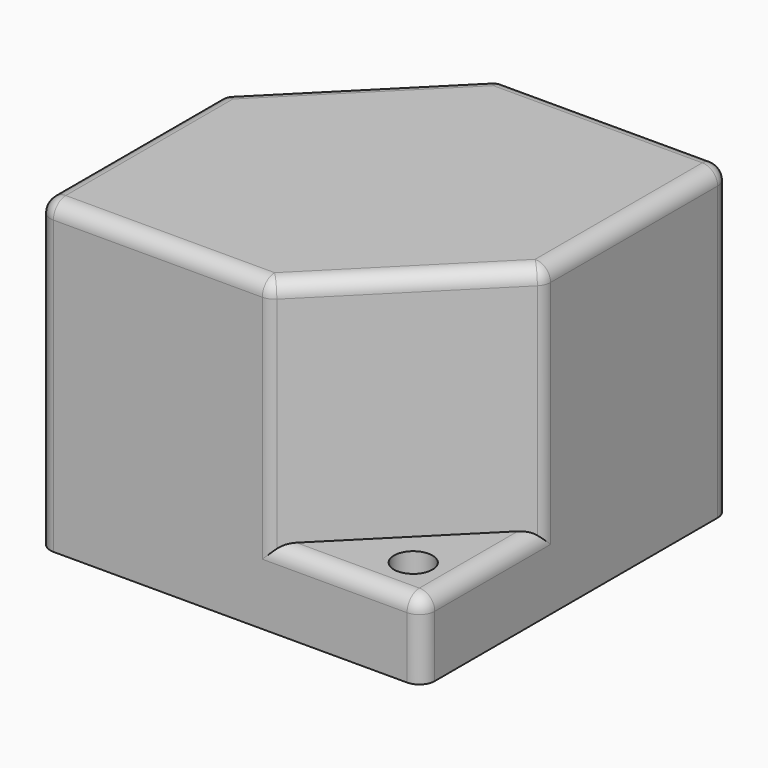
from build123d import *

# Parameters (mm, degrees)
F0_W     = 127
F0_H     = 127
F1_DEPTH = 101.6
F3_DEPTH = 76.2
F4_R     = 6.35
F5_DEPTH = 203.2
F6_T     = -2.54
F7_R     = 5.08


# Not quite as in the source:
# - a feature names something its author has since deleted; it is built from what else it names


with BuildPart() as f1:
    # F0 (on Top) → F1 (new body)
    with BuildSketch(Plane.XY):
        with Locations((2.0048860461, 1.4262827701)):
            Rectangle(F0_W, F0_H)
    extrude(amount=F1_DEPTH)

    # F2 (on face) → F3 (cut)
    with BuildSketch(Plane.XY.offset(101.6)):
        Polygon((-61.4951139539, 14.1262827701), (-10.6951139539, 64.9262827701), (-61.4951139539, 64.9262827701), align=None)
        Polygon((65.5048860461, -62.0737172299), (65.5048860461, -11.2737172299), (14.7048860461, -62.0737172299), align=None)
    extrude(amount=-F3_DEPTH, mode=Mode.SUBTRACT)

    # F4 (on face) → F5 (cut)
    with BuildSketch(Plane.XY.offset(25.4)):
        with Locations((-46.2551139539, 49.6862827701)):
            Circle(F4_R)
        with Locations((50.2648860461, -46.8337172299)):
            Circle(F4_R)
    extrude(amount=-F5_DEPTH, mode=Mode.SUBTRACT)

    # F6
    f6_openings = [f1.faces().sort_by_distance(p)[0] for p in [
        (2.004886, 1.426283, 0),
    ]]
    offset(amount=F6_T, openings=f6_openings, kind=Kind.INTERSECTION)

    # F7
    f7_edges = [f1.edges().sort_by_distance(p)[0] for p in [
        (-36.095114, 39.526283, 101.6),
        (-61.495114, -23.973717, 101.6),
        (-23.395114, -62.073717, 101.6),
        (27.404886, 64.926283, 101.6),
        (65.504886, 26.826283, 101.6),
        (40.104886, -36.673717, 101.6),
        (-61.495114, 14.126283, 63.5),
        (-10.695114, 64.926283, 63.5),
        (-61.495114, 39.526283, 25.4),
        (-36.095114, 64.926283, 25.4),
        (-61.495114, 64.926283, 12.7),
        (-61.495114, -62.073717, 50.8),
        (14.704886, -62.073717, 63.5),
        (65.504886, -11.273717, 63.5),
        (65.504886, -36.673717, 25.4),
        (40.104886, -62.073717, 25.4),
        (65.504886, -62.073717, 12.7),
        (65.504886, 64.926283, 50.8),
    ]]
    fillet(f7_edges, radius=F7_R)


solid = f1.part
